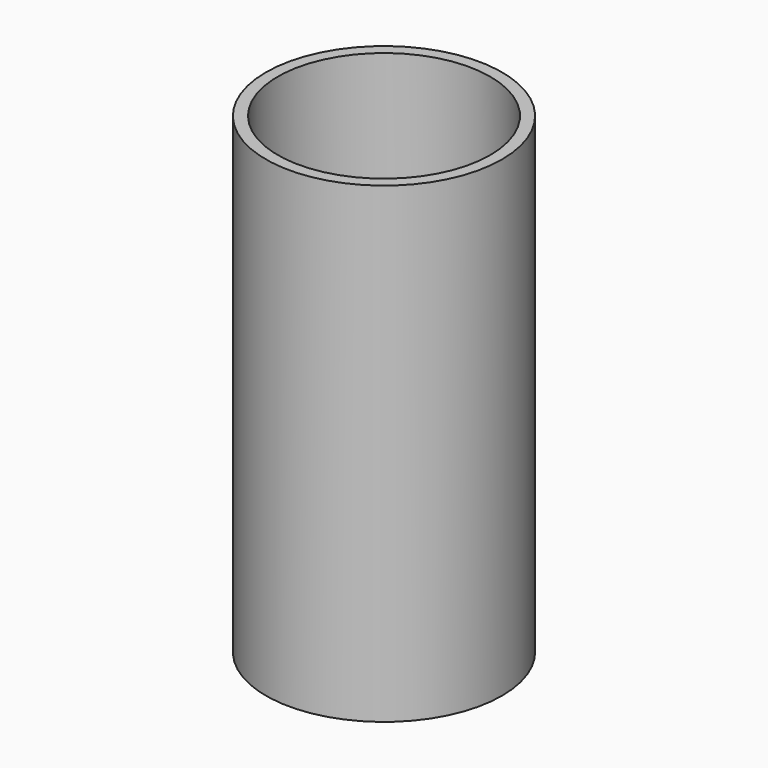
from build123d import *

# Parameters (mm, degrees)
F0_R     = 19.05
F1_DEPTH = 38.1
F3_R     = 16.129
F4_DEPTH = 22.86
F5_R     = 17.145
F6_DEPTH = 53.34


with BuildPart() as f1:
    # F0 (on Top) → F1 (new body, symmetric)
    with BuildSketch(Plane.XY):
        Circle(F0_R)
    extrude(amount=F1_DEPTH, both=True)

    # F3 (on face) → F4 (cut)
    with BuildSketch(Plane(origin=(0, 0, -38.1), x_dir=(1, 0, 0), z_dir=(0, 0, -1))):
        Circle(F3_R)
    extrude(amount=-F4_DEPTH, mode=Mode.SUBTRACT)

    # F5 (on face) → F6 (cut)
    with BuildSketch(Plane.XY.offset(38.1)):
        Circle(F5_R)
    extrude(amount=-F6_DEPTH, mode=Mode.SUBTRACT)


solid = f1.part
